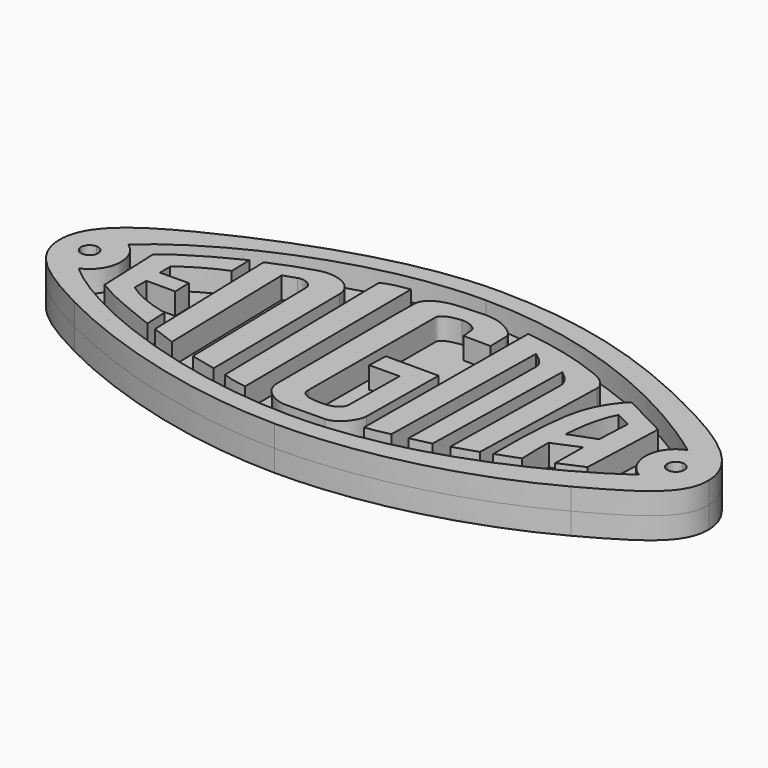
from build123d import *

# Parameters (mm, degrees)
F1_DEPTH = 1
F2_DEPTH = 1


# Not quite as in the source:
# - ends of sketch curves that miss each other by under 0.0002 mm in the source are joined


with BuildPart() as f1:
    # F0 (on Top) → F1 (new body)
    with BuildSketch(Plane.XY):
        with BuildLine():
            add(Edge.make_bspline(
                [(-14.9670643715, -0.1407183656), (-14.9569619615, 1.2571726483), (-13.641275343, 2.2858408304), (-11.5509025419, 3.3477109063)],
                knots=[0, 0, 0, 0, 1, 1, 1, 1], degree=3))
            add(Edge.make_bspline(
                [(-11.5044687858, -3.6532307803), (-13.8905338724, -2.4348834013), (-14.9771667815, -1.5386093795), (-14.9670643715, -0.1407183656)],
                knots=[0, 0, 0, 0, 1, 1, 1, 1], degree=3))
            add(Edge.make_bspline(
                [(0.0408589419, -6.5594502425), (-4.0268959211, -6.5322608085), (-8.2906712355, -5.2942260219), (-11.5044687858, -3.6532307803)],
                knots=[0, 0, 0, 0, 1, 1, 1, 1], degree=3))
            add(Edge.make_bspline(
                [(11.460803766, -3.7191493993), (8.3259909371, -5.4149417683), (4.1086135021, -6.5866396765), (0.0408589419, -6.5594502425)],
                knots=[0, 0, 0, 0, 1, 1, 1, 1], degree=3))
            add(Edge.make_bspline(
                [(15.0329356285, -0.2313463811), (15.0665385246, -1.6458235069), (13.7252402924, -2.4941911604), (11.460803766, -3.7191493993)],
                knots=[0, 0, 0, 0, 1, 1, 1, 1], degree=3))
            add(Edge.make_bspline(
                [(11.5176890114, 3.3904380032), (13.5946130245, 2.2916362132), (14.9993327324, 1.1831307446), (15.0329356285, -0.2313463811)],
                knots=[0, 0, 0, 0, 1, 1, 1, 1], degree=3))
            add(Edge.make_bspline(
                [(0.0012151267, 6.5835113531), (4.2558432307, 6.5477381404), (7.5924313242, 5.4671057322), (11.5176890114, 3.3904380032)],
                knots=[0, 0, 0, 0, 1, 1, 1, 1], degree=3))
            add(Edge.make_bspline(
                [(-11.5509025419, 3.3477109063), (-8.7841304286, 4.7531791819), (-4.2534132801, 6.6192845659), (0.0012151267, 6.5835113531)],
                knots=[0, 0, 0, 0, 1, 1, 1, 1], degree=3))
        make_face()
        with BuildLine():
            add(Edge.make_bspline(
                [(-13.6112109244, 0.2440781572), (-13.3944005743, 0.2441072219), (-13.2186146132, 0.0683763627), (-13.2185758603, -0.1484339874)],
                knots=[0, 0, 0, 0, 1, 1, 1, 1], degree=3))
            add(Edge.make_bspline(
                [(-13.2185758603, -0.1484339874), (-13.2185758603, -0.3653145773), (-13.3943303345, -0.5410769233), (-13.6111406847, -0.5410866115)],
                knots=[0, 0, 0, 0, 1, 1, 1, 1], degree=3))
            add(Edge.make_bspline(
                [(-13.6111406847, -0.5410866115), (-13.8279511862, -0.5410962997), (-14.0037212525, -0.3653498485), (-14.0037407803, -0.148539347)],
                knots=[0, 0, 0, 0, 1, 1, 1, 1], degree=3))
            add(Edge.make_bspline(
                [(-14.0037407803, -0.148539347), (-14.0037601568, 0.0682710031), (-13.8280214259, 0.2440490925), (-13.6112109244, 0.2440781572)],
                knots=[0, 0, 0, 0, 1, 1, 1, 1], degree=3))
        make_face(mode=Mode.SUBTRACT)
        with BuildLine():
            add(Edge.make_bspline(
                [(-0.0131874985, -5.7002234367), (-5.2648230774, -5.6636889404), (-10.8317908165, -3.4899332606), (-13.0370717195, -1.5029596918)],
                knots=[0, 0, 0, 0, 1, 1, 1, 1], degree=3))
            add(Edge.make_bspline(
                [(-13.0370717195, -1.5029596918), (-11.9503426849, -1.0492089526), (-11.8638049223, 0.4456897815), (-12.8094284057, 1.0703302885)],
                knots=[0, 0, 0, 0, 1, 1, 1, 1], degree=3))
            add(Edge.make_bspline(
                [(-12.8094284057, 1.0703302885), (-10.2644291395, 3.343872699), (-5.0939152955, 5.7284840957), (-0.0131874985, 5.7189015202)],
                knots=[0, 0, 0, 0, 1, 1, 1, 1], degree=3))
            add(Edge.make_bspline(
                [(-0.0131874985, 5.7189015202), (5.0675404498, 5.7093187933), (9.7327737855, 3.5101702421), (12.9692698175, 1.1270839859)],
                knots=[0, 0, 0, 0, 1, 1, 1, 1], degree=3))
            add(Edge.make_bspline(
                [(12.9692698175, 1.1270839859), (11.7931722383, 0.6908568469), (11.801028945, -0.9240995903), (12.8031188089, -1.4633658316)],
                knots=[0, 0, 0, 0, 1, 1, 1, 1], degree=3))
            add(Edge.make_bspline(
                [(12.8031188089, -1.4633658316), (10.1548959098, -3.3464114023), (5.2384480804, -5.7367579331), (-0.0131874985, -5.7002234367)],
                knots=[0, 0, 0, 0, 1, 1, 1, 1], degree=3))
        make_face(mode=Mode.SUBTRACT)
        with BuildLine():
            add(Edge.make_bspline(
                [(13.4484099464, 0.2319138177), (13.6652202965, 0.2319430338), (13.8410062576, 0.0562121746), (13.8410450105, -0.1605983269)],
                knots=[0, 0, 0, 0, 1, 1, 1, 1], degree=3))
            add(Edge.make_bspline(
                [(13.8410450105, -0.1605983269), (13.8410450105, -0.3774789168), (13.6652905362, -0.5532412628), (13.4484801861, -0.553250951)],
                knots=[0, 0, 0, 0, 1, 1, 1, 1], degree=3))
            add(Edge.make_bspline(
                [(13.4484801861, -0.553250951), (13.231669836, -0.5532606393), (13.0558996183, -0.3775140367), (13.0558802418, -0.1607036865)],
                knots=[0, 0, 0, 0, 1, 1, 1, 1], degree=3))
            add(Edge.make_bspline(
                [(13.0558802418, -0.1607036865), (13.055860714, 0.0561066636), (13.2315994449, 0.231884753), (13.4484099464, 0.2319138177)],
                knots=[0, 0, 0, 0, 1, 1, 1, 1], degree=3))
        make_face(mode=Mode.SUBTRACT)
    extrude(amount=F1_DEPTH)


with BuildPart() as f1b:
    # F0 (on Top) → F1, piece 2 (new body)
    with BuildSketch(Plane.XY):
        with BuildLine():
            Line((-11.6211207706, 1.0289036862), (-11.5002833157, -1.9165056063))
            add(Edge.make_bspline(
                [(-11.5002833157, -1.9165056063), (-10.5464697896, -2.5212275505), (-9.4578547276, -2.8833071235), (-8.4113801698, -3.3212389382)],
                knots=[0, 0, 0, 0, 1, 1, 1, 1], degree=3))
            Line((-8.4113801698, -3.3212389382), (-8.4566941776, -2.27146493))
            add(Edge.make_bspline(
                [(-8.4566941776, -2.27146493), (-9.605320607, -2.0319305152), (-10.5260527366, -1.4709255333), (-10.5260327546, -1.3651853806)],
                knots=[0, 0, 0, 0, 1, 1, 1, 1], degree=3))
            Line((-10.5260327546, -1.3651853806), (-10.5184803191, -0.7383417077))
            Line((-10.5184803191, -0.7383417077), (-9.189270283, -0.7383417077))
            Line((-9.189270283, -0.7383417077), (-9.2119272868, 0.0773099777))
            Line((-9.2119272868, 0.0773099777), (-10.5335851902, 0.0622055607))
            Line((-10.5335851902, 0.0622055607), (-10.5411371716, 0.6437347718))
            add(Edge.make_bspline(
                [(-10.5411371716, 0.6437347718), (-10.5413080782, 0.7288635012), (-9.4660527933, 1.4647343644), (-8.6001881822, 1.7841367955)],
                knots=[0, 0, 0, 0, 1, 1, 1, 1], degree=3))
            Line((-8.6001881822, 1.7841367955), (-8.6228450347, 2.8414632393))
            add(Edge.make_bspline(
                [(-8.6228450347, 2.8414632393), (-9.5944114998, 2.3620312522), (-10.7739830692, 1.7207511966), (-11.6211207706, 1.0289036862)],
                knots=[0, 0, 0, 0, 1, 1, 1, 1], degree=3))
        make_face()
    extrude(amount=F1_DEPTH)


with BuildPart() as f1c:
    # F0 (on Top) → F1, piece 3 (new body)
    with BuildSketch(Plane.XY):
        with BuildLine():
            Line((-4.3633304258, -4.5522689775), (-4.4388534188, 2.788596796))
            add(Edge.make_bspline(
                [(-4.4388534188, 2.788596796), (-4.4690630096, 3.6797719285), (-5.5116984517, 3.9135012722), (-6.100366683, 3.7704002467)],
                knots=[0, 0, 0, 0, 1, 1, 1, 1], degree=3))
            add(Edge.make_bspline(
                [(-8.1243912523, 3.0302717058), (-7.7536792271, 3.1870081507), (-7.0454069014, 3.486464545), (-6.4053945164, 3.6787551609), (-6.100366683, 3.7704002467)],
                knots=[0, 0, 0, 0, 0.5234032331, 1, 1, 1, 1], degree=3))
            Line((-8.1243912523, 3.0302717058), (-7.9280308043, -3.4798379654))
            Line((-7.9280308043, -3.4798379654), (-6.8253903528, -3.8876641865))
            Line((-6.8253903528, -3.8876641865), (-6.976436793, 2.6375503558))
            Line((-6.976436793, 2.6375503558), (-6.4024595634, 2.8339108037))
            add(Edge.make_bspline(
                [(-6.4024595634, 2.8339108037), (-6.1154712513, 2.9396436903), (-5.707645333, 2.7281783713), (-5.692540916, 2.4713988931)],
                knots=[0, 0, 0, 0, 1, 1, 1, 1], degree=3))
            Line((-5.692540916, 2.4713988931), (-5.5414940217, -4.2803850824))
            Line((-5.5414940217, -4.2803850824), (-4.3633304258, -4.5522689775))
        make_face()
    extrude(amount=F1_DEPTH)


with BuildPart() as f1d:
    # F0 (on Top) → F1, piece 4 (new body)
    with BuildSketch(Plane.XY):
        with BuildLine():
            Line((-2.5960847291, -4.9449901761), (-2.6565033052, 4.6917845159))
            add(Edge.make_bspline(
                [(-2.6565033052, 4.6917845159), (-3.0422194537, 4.6081617018), (-3.313422296, 4.6390521941), (-3.8799812116, 4.374586613)],
                knots=[0, 0, 0, 0, 1, 1, 1, 1], degree=3))
            Line((-3.8799812116, 4.374586613), (-3.7289343173, -4.6882113035))
            add(Edge.make_bspline(
                [(-3.7289343173, -4.6882113035), (-3.2986876972, -4.852749069), (-2.9477797221, -4.8982792456), (-2.5960847291, -4.9449901761)],
                knots=[0, 0, 0, 0, 1, 1, 1, 1], degree=3))
        make_face()
    extrude(amount=F1_DEPTH)


with BuildPart() as f1e:
    # F0 (on Top) → F1, piece 5 (new body)
    with BuildSketch(Plane.XY):
        with BuildLine():
            Line((1.2556039615, -0.8516265756), (1.2253949763, -3.6913037385))
            add(Edge.make_bspline(
                [(1.2253949763, -3.6913037385), (1.2253945221, -3.9782917478), (1.0288969251, -4.2504746159), (0.3191149727, -4.2501756429)],
                knots=[0, 0, 0, 0, 1, 1, 1, 1], degree=3))
            add(Edge.make_bspline(
                [(0.3191149727, -4.2501756429), (-0.4969122832, -4.2498338298), (-0.6475831528, -4.0085011873), (-0.6324787359, -3.7366172921)],
                knots=[0, 0, 0, 0, 1, 1, 1, 1], degree=3))
            add(Edge.make_bspline(
                [(-0.6324787359, -3.7366172921), (-0.6173741676, -3.464733397), (-0.6022691451, 3.2719461615), (-0.6022691451, 3.5438299052)],
                knots=[0, 0, 0, 0, 1, 1, 1, 1], degree=3))
            add(Edge.make_bspline(
                [(-0.6022691451, 3.5438299052), (-0.6022691451, 3.8157138003), (-0.0433969379, 3.9516558236), (0.288905836, 3.9667606946)],
                knots=[0, 0, 0, 0, 1, 1, 1, 1], degree=3))
            add(Edge.make_bspline(
                [(0.288905836, 3.9667606946), (0.6212083072, 3.981865263), (1.0441390966, 3.7724048037), (1.0441390966, 3.5438299052)],
                knots=[0, 0, 0, 0, 1, 1, 1, 1], degree=3))
            Line((1.0441390966, 3.5438299052), (1.089452953, 3.0453761227))
            Line((1.089452953, 3.0453761227), (2.3431399961, 3.0302717058))
            Line((2.3431399961, 3.0302717058), (2.3280349736, 3.9516558236))
            add(Edge.make_bspline(
                [(2.3280349736, 3.9516558236), (2.3129305567, 4.2839585975), (1.6030113038, 4.7068889328), (1.089452953, 4.78241238)],
                knots=[0, 0, 0, 0, 1, 1, 1, 1], degree=3))
            add(Edge.make_bspline(
                [(1.089452953, 4.78241238), (0.5758942995, 4.8579358271), (0.54568486, 4.78241238), (-0.2699668253, 4.767307963)],
                knots=[0, 0, 0, 0, 1, 1, 1, 1], degree=3))
            add(Edge.make_bspline(
                [(-0.2699668253, 4.767307963), (-1.0856185106, 4.7522029406), (-1.7955376121, 4.4803190454), (-1.8559561882, 3.9365512552)],
                knots=[0, 0, 0, 0, 1, 1, 1, 1], degree=3))
            add(Edge.make_bspline(
                [(-1.8559561882, 3.9365512552), (-1.916375067, 3.392783465), (-1.8106421804, -3.4345239576), (-1.8408516199, -4.053815195)],
                knots=[0, 0, 0, 0, 1, 1, 1, 1], degree=3))
            add(Edge.make_bspline(
                [(-1.8408516199, -4.053815195), (-1.8710610593, -4.673106281), (-1.1007233817, -5.1564556465), (-0.5871647281, -5.1564556465)],
                knots=[0, 0, 0, 0, 1, 1, 1, 1], degree=3))
            add(Edge.make_bspline(
                [(-0.5871647281, -5.1564556465), (-0.0736059232, -5.1564556465), (0.6967317544, -5.1564556465), (1.2556039615, -5.1413510782)],
                knots=[0, 0, 0, 0, 1, 1, 1, 1], degree=3))
            add(Edge.make_bspline(
                [(1.2556039615, -5.1413510782), (1.8144767742, -5.1262462071), (2.2676165489, -4.4465363936), (2.2827211173, -4.0387106267)],
                knots=[0, 0, 0, 0, 1, 1, 1, 1], degree=3))
            Line((2.2827211173, -4.0387106267), (2.3280349736, 0.0546529738))
            Line((2.3280349736, 0.0546529738), (-0.1038153626, 0.0546529738))
            Line((-0.1038153626, 0.0546529738), (-0.1340249534, -0.8667315981))
            Line((-0.1340249534, -0.8667315981), (1.2556039615, -0.8516265756))
        make_face()
    extrude(amount=F1_DEPTH)


with BuildPart() as f1f:
    # F0 (on Top) → F1, piece 6 (new body)
    with BuildSketch(Plane.XY):
        with BuildLine():
            Line((7.2068412741, -3.661093845), (7.4032021762, 2.849015372))
            add(Edge.make_bspline(
                [(7.4032021762, 2.849015372), (7.4183067446, 3.1511087066), (7.049798723, 3.505934817), (6.5875500368, 3.6797719285)],
                knots=[0, 0, 0, 0, 1, 1, 1, 1], degree=3))
            ThreePointArc((6.5875500368, 3.6797719285), (4.731040618, 4.2753288203), (2.8113843392, 4.6162613714))
            Line((2.8113843392, 4.6162613714), (2.7509657631, -4.778839319))
            add(Edge.make_bspline(
                [(2.7509657631, -4.778839319), (3.1297758632, -4.7196140613), (3.5135646579, -4.6653676496), (3.8536062146, -4.5673738486)],
                knots=[0, 0, 0, 0, 1, 1, 1, 1], degree=3))
            Line((3.8536062146, -4.5673738486), (4.0046528062, 3.5891443671))
            add(Edge.make_bspline(
                [(4.0046528062, 3.5891443671), (4.0720203225, 3.5379805902), (4.1828123319, 3.4522951468), (4.2144659213, 3.4274451231), (4.2906508935, 3.3664320253), (4.4687473777, 3.2021661464), (4.6033155082, 2.9884969513), (4.6326551395, 2.8839476867), (4.6373056055, 2.824720552), (4.6390484605, 2.8037018184)],
                knots=[0, 0, 0, 0, 0.1850054035, 0.2612916033, 0.3753300897, 0.5703100306, 0.7666527828, 0.8936191452, 1, 1, 1, 1], degree=3))
            Line((4.6390484605, 2.8037018184), (4.5333160281, -4.4314319767))
            add(Edge.make_bspline(
                [(4.5333160281, -4.4314319767), (4.8354789968, -4.3709433123), (5.1293064479, -4.318790771), (5.4698050169, -4.2199665063)],
                knots=[0, 0, 0, 0, 1, 1, 1, 1], degree=3))
            Line((5.4698050169, -4.2199665063), (5.6359564796, 3.0604806911))
            add(Edge.make_bspline(
                [(5.6359564796, 3.0604806911), (5.785887239, 2.9409553318), (6.0576444833, 2.7243094457), (6.2258203773, 2.3756907044), (6.2361157634, 2.2599070967), (6.2401426945, 2.2146195663)],
                knots=[0, 0, 0, 0, 0.4283490631, 0.7764047978, 1, 1, 1, 1], degree=3))
            Line((6.2401426945, 2.2146195663), (6.119305391, -4.0085011873))
            add(Edge.make_bspline(
                [(6.119305391, -4.0085011873), (6.4699454257, -3.904570767), (6.817240445, -3.8039850596), (7.2068412741, -3.661093845)],
                knots=[0, 0, 0, 0, 1, 1, 1, 1], degree=3))
        make_face()
    extrude(amount=F1_DEPTH)


with BuildPart() as f1g:
    # F0 (on Top) → F1, piece 7 (new body)
    with BuildSketch(Plane.XY):
        with BuildLine():
            Line((9.8671853699, -2.6448491628), (10.9779687853, -2.164221738))
            Line((10.9779687853, -2.164221738), (11.1274973511, 1.7128389338))
            Line((11.1274973511, 1.7128389338), (9.055459086, 2.7808999451))
            add(Edge.make_bspline(
                [(7.6776605692, -3.4779368001), (7.6761910448, -2.9670023712), (7.6730666864, -1.8807037051), (7.7992836376, 0.1813668207), (8.0436769948, 1.2326744215), (8.4274407257, 2.0619125257), (8.9246206003, 2.6759028048), (9.0247880348, 2.756286601), (9.055459086, 2.7808999451)],
                knots=[0, 0, 0, 0, 0.2136285367, 0.4541960402, 0.628207252, 0.7899148708, 0.935672389, 1, 1, 1, 1], degree=3))
            Line((7.6776605692, -3.4779368001), (8.7136795503, -3.1041153856))
            add(Edge.make_bspline(
                [(8.7136795503, -3.1041153856), (8.7045593073, -2.8555582906), (8.6868684619, -2.3734236481), (8.6852845097, -1.6678730588), (8.6948580771, -1.5618086592), (8.7015062661, -1.5565972505), (8.702999025, -1.5554271008)],
                knots=[0, 0, 0, 0, 0.4262627423, 0.8268363249, 0.9611184917, 1, 1, 1, 1], degree=3))
            Line((8.702999025, -1.5554271008), (9.8885467233, -1.0534384739))
            Line((9.8885467233, -1.0534384739), (9.8671853699, -2.6448491628))
        make_face()
        with BuildLine():
            add(Edge.make_bspline(
                [(9.3011131368, 1.7235196105), (8.9318485244, 0.9931556023), (8.8098038243, 0.1356684408), (8.7564021058, -0.6475751806)],
                knots=[0, 0, 0, 0, 1, 1, 1, 1], degree=3))
            Line((9.3011131368, 1.7235196105), (10.0167139357, 1.3603788727))
            Line((10.0167139357, 1.3603788727), (9.9419496528, -0.1989896346))
            Line((9.9419496528, -0.1989896346), (8.7564021058, -0.6475751806))
        make_face(mode=Mode.SUBTRACT)
    extrude(amount=F1_DEPTH)


with BuildPart() as f2:
    # F0 (on Top) → F2 (new body)
    with BuildSketch(Plane.XY):
        with BuildLine():
            add(Edge.make_bspline(
                [(-14.9670643715, -0.1407183656), (-14.9569619615, 1.2571726483), (-13.641275343, 2.2858408304), (-11.5509025419, 3.3477109063)],
                knots=[0, 0, 0, 0, 1, 1, 1, 1], degree=3))
            add(Edge.make_bspline(
                [(-11.5044687858, -3.6532307803), (-13.8905338724, -2.4348834013), (-14.9771667815, -1.5386093795), (-14.9670643715, -0.1407183656)],
                knots=[0, 0, 0, 0, 1, 1, 1, 1], degree=3))
            add(Edge.make_bspline(
                [(0.0408589419, -6.5594502425), (-4.0268959211, -6.5322608085), (-8.2906712355, -5.2942260219), (-11.5044687858, -3.6532307803)],
                knots=[0, 0, 0, 0, 1, 1, 1, 1], degree=3))
            add(Edge.make_bspline(
                [(11.460803766, -3.7191493993), (8.3259909371, -5.4149417683), (4.1086135021, -6.5866396765), (0.0408589419, -6.5594502425)],
                knots=[0, 0, 0, 0, 1, 1, 1, 1], degree=3))
            add(Edge.make_bspline(
                [(15.0329356285, -0.2313463811), (15.0665385246, -1.6458235069), (13.7252402924, -2.4941911604), (11.460803766, -3.7191493993)],
                knots=[0, 0, 0, 0, 1, 1, 1, 1], degree=3))
            add(Edge.make_bspline(
                [(11.5176890114, 3.3904380032), (13.5946130245, 2.2916362132), (14.9993327324, 1.1831307446), (15.0329356285, -0.2313463811)],
                knots=[0, 0, 0, 0, 1, 1, 1, 1], degree=3))
            add(Edge.make_bspline(
                [(0.0012151267, 6.5835113531), (4.2558432307, 6.5477381404), (7.5924313242, 5.4671057322), (11.5176890114, 3.3904380032)],
                knots=[0, 0, 0, 0, 1, 1, 1, 1], degree=3))
            add(Edge.make_bspline(
                [(-11.5509025419, 3.3477109063), (-8.7841304286, 4.7531791819), (-4.2534132801, 6.6192845659), (0.0012151267, 6.5835113531)],
                knots=[0, 0, 0, 0, 1, 1, 1, 1], degree=3))
        make_face()
        with BuildLine():
            add(Edge.make_bspline(
                [(-13.6112109244, 0.2440781572), (-13.3944005743, 0.2441072219), (-13.2186146132, 0.0683763627), (-13.2185758603, -0.1484339874)],
                knots=[0, 0, 0, 0, 1, 1, 1, 1], degree=3))
            add(Edge.make_bspline(
                [(-13.2185758603, -0.1484339874), (-13.2185758603, -0.3653145773), (-13.3943303345, -0.5410769233), (-13.6111406847, -0.5410866115)],
                knots=[0, 0, 0, 0, 1, 1, 1, 1], degree=3))
            add(Edge.make_bspline(
                [(-13.6111406847, -0.5410866115), (-13.8279511862, -0.5410962997), (-14.0037212525, -0.3653498485), (-14.0037407803, -0.148539347)],
                knots=[0, 0, 0, 0, 1, 1, 1, 1], degree=3))
            add(Edge.make_bspline(
                [(-14.0037407803, -0.148539347), (-14.0037601568, 0.0682710031), (-13.8280214259, 0.2440490925), (-13.6112109244, 0.2440781572)],
                knots=[0, 0, 0, 0, 1, 1, 1, 1], degree=3))
        make_face(mode=Mode.SUBTRACT)
        with BuildLine():
            add(Edge.make_bspline(
                [(-0.0131874985, -5.7002234367), (-5.2648230774, -5.6636889404), (-10.8317908165, -3.4899332606), (-13.0370717195, -1.5029596918)],
                knots=[0, 0, 0, 0, 1, 1, 1, 1], degree=3))
            add(Edge.make_bspline(
                [(-13.0370717195, -1.5029596918), (-11.9503426849, -1.0492089526), (-11.8638049223, 0.4456897815), (-12.8094284057, 1.0703302885)],
                knots=[0, 0, 0, 0, 1, 1, 1, 1], degree=3))
            add(Edge.make_bspline(
                [(-12.8094284057, 1.0703302885), (-10.2644291395, 3.343872699), (-5.0939152955, 5.7284840957), (-0.0131874985, 5.7189015202)],
                knots=[0, 0, 0, 0, 1, 1, 1, 1], degree=3))
            add(Edge.make_bspline(
                [(-0.0131874985, 5.7189015202), (5.0675404498, 5.7093187933), (9.7327737855, 3.5101702421), (12.9692698175, 1.1270839859)],
                knots=[0, 0, 0, 0, 1, 1, 1, 1], degree=3))
            add(Edge.make_bspline(
                [(12.9692698175, 1.1270839859), (11.7931722383, 0.6908568469), (11.801028945, -0.9240995903), (12.8031188089, -1.4633658316)],
                knots=[0, 0, 0, 0, 1, 1, 1, 1], degree=3))
            add(Edge.make_bspline(
                [(12.8031188089, -1.4633658316), (10.1548959098, -3.3464114023), (5.2384480804, -5.7367579331), (-0.0131874985, -5.7002234367)],
                knots=[0, 0, 0, 0, 1, 1, 1, 1], degree=3))
        make_face(mode=Mode.SUBTRACT)
        with BuildLine():
            add(Edge.make_bspline(
                [(13.4484099464, 0.2319138177), (13.6652202965, 0.2319430338), (13.8410062576, 0.0562121746), (13.8410450105, -0.1605983269)],
                knots=[0, 0, 0, 0, 1, 1, 1, 1], degree=3))
            add(Edge.make_bspline(
                [(13.8410450105, -0.1605983269), (13.8410450105, -0.3774789168), (13.6652905362, -0.5532412628), (13.4484801861, -0.553250951)],
                knots=[0, 0, 0, 0, 1, 1, 1, 1], degree=3))
            add(Edge.make_bspline(
                [(13.4484801861, -0.553250951), (13.231669836, -0.5532606393), (13.0558996183, -0.3775140367), (13.0558802418, -0.1607036865)],
                knots=[0, 0, 0, 0, 1, 1, 1, 1], degree=3))
            add(Edge.make_bspline(
                [(13.0558802418, -0.1607036865), (13.055860714, 0.0561066636), (13.2315994449, 0.231884753), (13.4484099464, 0.2319138177)],
                knots=[0, 0, 0, 0, 1, 1, 1, 1], degree=3))
        make_face(mode=Mode.SUBTRACT)
        with BuildLine():
            add(Edge.make_bspline(
                [(-13.0370717195, -1.5029596918), (-11.9503426849, -1.0492089526), (-11.8638049223, 0.4456897815), (-12.8094284057, 1.0703302885)],
                knots=[0, 0, 0, 0, 1, 1, 1, 1], degree=3))
            add(Edge.make_bspline(
                [(-0.0131874985, -5.7002234367), (-5.2648230774, -5.6636889404), (-10.8317908165, -3.4899332606), (-13.0370717195, -1.5029596918)],
                knots=[0, 0, 0, 0, 1, 1, 1, 1], degree=3))
            add(Edge.make_bspline(
                [(12.8031188089, -1.4633658316), (10.1548959098, -3.3464114023), (5.2384480804, -5.7367579331), (-0.0131874985, -5.7002234367)],
                knots=[0, 0, 0, 0, 1, 1, 1, 1], degree=3))
            add(Edge.make_bspline(
                [(12.9692698175, 1.1270839859), (11.7931722383, 0.6908568469), (11.801028945, -0.9240995903), (12.8031188089, -1.4633658316)],
                knots=[0, 0, 0, 0, 1, 1, 1, 1], degree=3))
            add(Edge.make_bspline(
                [(-0.0131874985, 5.7189015202), (5.0675404498, 5.7093187933), (9.7327737855, 3.5101702421), (12.9692698175, 1.1270839859)],
                knots=[0, 0, 0, 0, 1, 1, 1, 1], degree=3))
            add(Edge.make_bspline(
                [(-12.8094284057, 1.0703302885), (-10.2644291395, 3.343872699), (-5.0939152955, 5.7284840957), (-0.0131874985, 5.7189015202)],
                knots=[0, 0, 0, 0, 1, 1, 1, 1], degree=3))
        make_face()
        with BuildLine():
            add(Edge.make_bspline(
                [(-11.5002833157, -1.9165056063), (-10.5464697896, -2.5212275505), (-9.4578547276, -2.8833071235), (-8.4113801698, -3.3212389382)],
                knots=[0, 0, 0, 0, 1, 1, 1, 1], degree=3))
            Line((-11.5002833157, -1.9165056063), (-11.6211207706, 1.0289036862))
            add(Edge.make_bspline(
                [(-8.6228450347, 2.8414632393), (-9.5944114998, 2.3620312522), (-10.7739830692, 1.7207511966), (-11.6211207706, 1.0289036862)],
                knots=[0, 0, 0, 0, 1, 1, 1, 1], degree=3))
            Line((-8.6228450347, 2.8414632393), (-8.6001881822, 1.7841367955))
            add(Edge.make_bspline(
                [(-10.5411371716, 0.6437347718), (-10.5413080782, 0.7288635012), (-9.4660527933, 1.4647343644), (-8.6001881822, 1.7841367955)],
                knots=[0, 0, 0, 0, 1, 1, 1, 1], degree=3))
            Line((-10.5411371716, 0.6437347718), (-10.5335851902, 0.0622055607))
            Line((-10.5335851902, 0.0622055607), (-9.2119272868, 0.0773099777))
            Line((-9.2119272868, 0.0773099777), (-9.189270283, -0.7383417077))
            Line((-9.189270283, -0.7383417077), (-10.5184803191, -0.7383417077))
            Line((-10.5184803191, -0.7383417077), (-10.5260327546, -1.3651853806))
            add(Edge.make_bspline(
                [(-8.4566941776, -2.27146493), (-9.605320607, -2.0319305152), (-10.5260527366, -1.4709255333), (-10.5260327546, -1.3651853806)],
                knots=[0, 0, 0, 0, 1, 1, 1, 1], degree=3))
            Line((-8.4566941776, -2.27146493), (-8.4113801698, -3.3212389382))
        make_face(mode=Mode.SUBTRACT)
        with BuildLine():
            add(Edge.make_bspline(
                [(-4.4388534188, 2.788596796), (-4.4690630096, 3.6797719285), (-5.5116984517, 3.9135012722), (-6.100366683, 3.7704002467)],
                knots=[0, 0, 0, 0, 1, 1, 1, 1], degree=3))
            Line((-4.4388534188, 2.788596796), (-4.3633304258, -4.5522689775))
            Line((-4.3633304258, -4.5522689775), (-5.5414940217, -4.2803850824))
            Line((-5.5414940217, -4.2803850824), (-5.692540916, 2.4713988931))
            add(Edge.make_bspline(
                [(-6.4024595634, 2.8339108037), (-6.1154712513, 2.9396436903), (-5.707645333, 2.7281783713), (-5.692540916, 2.4713988931)],
                knots=[0, 0, 0, 0, 1, 1, 1, 1], degree=3))
            Line((-6.4024595634, 2.8339108037), (-6.976436793, 2.6375503558))
            Line((-6.976436793, 2.6375503558), (-6.8253903528, -3.8876641865))
            Line((-6.8253903528, -3.8876641865), (-7.9280308043, -3.4798379654))
            Line((-7.9280308043, -3.4798379654), (-8.1243912523, 3.0302717058))
            add(Edge.make_bspline(
                [(-8.1243912523, 3.0302717058), (-7.7536792271, 3.1870081507), (-7.0454069014, 3.486464545), (-6.4053945164, 3.6787551609), (-6.100366683, 3.7704002467)],
                knots=[0, 0, 0, 0, 0.5234032331, 1, 1, 1, 1], degree=3))
        make_face(mode=Mode.SUBTRACT)
        with BuildLine():
            add(Edge.make_bspline(
                [(-2.6565033052, 4.6917845159), (-3.0422194537, 4.6081617018), (-3.313422296, 4.6390521941), (-3.8799812116, 4.374586613)],
                knots=[0, 0, 0, 0, 1, 1, 1, 1], degree=3))
            Line((-2.6565033052, 4.6917845159), (-2.5960847291, -4.9449901761))
            add(Edge.make_bspline(
                [(-3.7289343173, -4.6882113035), (-3.2986876972, -4.852749069), (-2.9477797221, -4.8982792456), (-2.5960847291, -4.9449901761)],
                knots=[0, 0, 0, 0, 1, 1, 1, 1], degree=3))
            Line((-3.7289343173, -4.6882113035), (-3.8799812116, 4.374586613))
        make_face(mode=Mode.SUBTRACT)
        with BuildLine():
            add(Edge.make_bspline(
                [(1.2253949763, -3.6913037385), (1.2253945221, -3.9782917478), (1.0288969251, -4.2504746159), (0.3191149727, -4.2501756429)],
                knots=[0, 0, 0, 0, 1, 1, 1, 1], degree=3))
            Line((1.2253949763, -3.6913037385), (1.2556039615, -0.8516265756))
            Line((1.2556039615, -0.8516265756), (-0.1340249534, -0.8667315981))
            Line((-0.1340249534, -0.8667315981), (-0.1038153626, 0.0546529738))
            Line((-0.1038153626, 0.0546529738), (2.3280349736, 0.0546529738))
            Line((2.3280349736, 0.0546529738), (2.2827211173, -4.0387106267))
            add(Edge.make_bspline(
                [(1.2556039615, -5.1413510782), (1.8144767742, -5.1262462071), (2.2676165489, -4.4465363936), (2.2827211173, -4.0387106267)],
                knots=[0, 0, 0, 0, 1, 1, 1, 1], degree=3))
            add(Edge.make_bspline(
                [(-0.5871647281, -5.1564556465), (-0.0736059232, -5.1564556465), (0.6967317544, -5.1564556465), (1.2556039615, -5.1413510782)],
                knots=[0, 0, 0, 0, 1, 1, 1, 1], degree=3))
            add(Edge.make_bspline(
                [(-1.8408516199, -4.053815195), (-1.8710610593, -4.673106281), (-1.1007233817, -5.1564556465), (-0.5871647281, -5.1564556465)],
                knots=[0, 0, 0, 0, 1, 1, 1, 1], degree=3))
            add(Edge.make_bspline(
                [(-1.8559561882, 3.9365512552), (-1.916375067, 3.392783465), (-1.8106421804, -3.4345239576), (-1.8408516199, -4.053815195)],
                knots=[0, 0, 0, 0, 1, 1, 1, 1], degree=3))
            add(Edge.make_bspline(
                [(-0.2699668253, 4.767307963), (-1.0856185106, 4.7522029406), (-1.7955376121, 4.4803190454), (-1.8559561882, 3.9365512552)],
                knots=[0, 0, 0, 0, 1, 1, 1, 1], degree=3))
            add(Edge.make_bspline(
                [(1.089452953, 4.78241238), (0.5758942995, 4.8579358271), (0.54568486, 4.78241238), (-0.2699668253, 4.767307963)],
                knots=[0, 0, 0, 0, 1, 1, 1, 1], degree=3))
            add(Edge.make_bspline(
                [(2.3280349736, 3.9516558236), (2.3129305567, 4.2839585975), (1.6030113038, 4.7068889328), (1.089452953, 4.78241238)],
                knots=[0, 0, 0, 0, 1, 1, 1, 1], degree=3))
            Line((2.3280349736, 3.9516558236), (2.3431399961, 3.0302717058))
            Line((2.3431399961, 3.0302717058), (1.089452953, 3.0453761227))
            Line((1.089452953, 3.0453761227), (1.0441390966, 3.5438299052))
            add(Edge.make_bspline(
                [(0.288905836, 3.9667606946), (0.6212083072, 3.981865263), (1.0441390966, 3.7724048037), (1.0441390966, 3.5438299052)],
                knots=[0, 0, 0, 0, 1, 1, 1, 1], degree=3))
            add(Edge.make_bspline(
                [(-0.6022691451, 3.5438299052), (-0.6022691451, 3.8157138003), (-0.0433969379, 3.9516558236), (0.288905836, 3.9667606946)],
                knots=[0, 0, 0, 0, 1, 1, 1, 1], degree=3))
            add(Edge.make_bspline(
                [(-0.6324787359, -3.7366172921), (-0.6173741676, -3.464733397), (-0.6022691451, 3.2719461615), (-0.6022691451, 3.5438299052)],
                knots=[0, 0, 0, 0, 1, 1, 1, 1], degree=3))
            add(Edge.make_bspline(
                [(0.3191149727, -4.2501756429), (-0.4969122832, -4.2498338298), (-0.6475831528, -4.0085011873), (-0.6324787359, -3.7366172921)],
                knots=[0, 0, 0, 0, 1, 1, 1, 1], degree=3))
        make_face(mode=Mode.SUBTRACT)
        with BuildLine():
            add(Edge.make_bspline(
                [(7.4032021762, 2.849015372), (7.4183067446, 3.1511087066), (7.049798723, 3.505934817), (6.5875500368, 3.6797719285)],
                knots=[0, 0, 0, 0, 1, 1, 1, 1], degree=3))
            Line((7.4032021762, 2.849015372), (7.2068412741, -3.661093845))
            add(Edge.make_bspline(
                [(6.119305391, -4.0085011873), (6.4699454257, -3.904570767), (6.817240445, -3.8039850596), (7.2068412741, -3.661093845)],
                knots=[0, 0, 0, 0, 1, 1, 1, 1], degree=3))
            Line((6.119305391, -4.0085011873), (6.2401426945, 2.2146195663))
            add(Edge.make_bspline(
                [(5.6359564796, 3.0604806911), (5.785887239, 2.9409553318), (6.0576444833, 2.7243094457), (6.2258203773, 2.3756907044), (6.2361157634, 2.2599070967), (6.2401426945, 2.2146195663)],
                knots=[0, 0, 0, 0, 0.4283490631, 0.7764047978, 1, 1, 1, 1], degree=3))
            Line((5.6359564796, 3.0604806911), (5.4698050169, -4.2199665063))
            add(Edge.make_bspline(
                [(4.5333160281, -4.4314319767), (4.8354789968, -4.3709433123), (5.1293064479, -4.318790771), (5.4698050169, -4.2199665063)],
                knots=[0, 0, 0, 0, 1, 1, 1, 1], degree=3))
            Line((4.5333160281, -4.4314319767), (4.6390484605, 2.8037018184))
            add(Edge.make_bspline(
                [(4.0046528062, 3.5891443671), (4.0720203225, 3.5379805902), (4.1828123319, 3.4522951468), (4.2144659213, 3.4274451231), (4.2906508935, 3.3664320253), (4.4687473777, 3.2021661464), (4.6033155082, 2.9884969513), (4.6326551395, 2.8839476867), (4.6373056055, 2.824720552), (4.6390484605, 2.8037018184)],
                knots=[0, 0, 0, 0, 0.1850054035, 0.2612916033, 0.3753300897, 0.5703100306, 0.7666527828, 0.8936191452, 1, 1, 1, 1], degree=3))
            Line((4.0046528062, 3.5891443671), (3.8536062146, -4.5673738486))
            add(Edge.make_bspline(
                [(2.7509657631, -4.778839319), (3.1297758632, -4.7196140613), (3.5135646579, -4.6653676496), (3.8536062146, -4.5673738486)],
                knots=[0, 0, 0, 0, 1, 1, 1, 1], degree=3))
            Line((2.7509657631, -4.778839319), (2.8113843392, 4.6162613714))
            ThreePointArc((2.8113843392, 4.6162613714), (4.731040618, 4.2753288203), (6.5875500368, 3.6797719285))
        make_face(mode=Mode.SUBTRACT)
        with BuildLine():
            Line((11.1274973511, 1.7128389338), (10.9779687853, -2.164221738))
            Line((10.9779687853, -2.164221738), (9.8671853699, -2.6448491628))
            Line((9.8671853699, -2.6448491628), (9.8885467233, -1.0534384739))
            Line((9.8885467233, -1.0534384739), (8.702999025, -1.5554271008))
            add(Edge.make_bspline(
                [(8.7136795503, -3.1041153856), (8.7045593073, -2.8555582906), (8.6868684619, -2.3734236481), (8.6852845097, -1.6678730588), (8.6948580771, -1.5618086592), (8.7015062661, -1.5565972505), (8.702999025, -1.5554271008)],
                knots=[0, 0, 0, 0, 0.4262627423, 0.8268363249, 0.9611184917, 1, 1, 1, 1], degree=3))
            Line((8.7136795503, -3.1041153856), (7.6776605692, -3.4779368001))
            add(Edge.make_bspline(
                [(7.6776605692, -3.4779368001), (7.6761910448, -2.9670023712), (7.6730666864, -1.8807037051), (7.7992836376, 0.1813668207), (8.0436769948, 1.2326744215), (8.4274407257, 2.0619125257), (8.9246206003, 2.6759028048), (9.0247880348, 2.756286601), (9.055459086, 2.7808999451)],
                knots=[0, 0, 0, 0, 0.2136285367, 0.4541960402, 0.628207252, 0.7899148708, 0.935672389, 1, 1, 1, 1], degree=3))
            Line((9.055459086, 2.7808999451), (11.1274973511, 1.7128389338))
        make_face(mode=Mode.SUBTRACT)
        with BuildLine():
            Line((-11.6211207706, 1.0289036862), (-11.5002833157, -1.9165056063))
            add(Edge.make_bspline(
                [(-11.5002833157, -1.9165056063), (-10.5464697896, -2.5212275505), (-9.4578547276, -2.8833071235), (-8.4113801698, -3.3212389382)],
                knots=[0, 0, 0, 0, 1, 1, 1, 1], degree=3))
            Line((-8.4113801698, -3.3212389382), (-8.4566941776, -2.27146493))
            add(Edge.make_bspline(
                [(-8.4566941776, -2.27146493), (-9.605320607, -2.0319305152), (-10.5260527366, -1.4709255333), (-10.5260327546, -1.3651853806)],
                knots=[0, 0, 0, 0, 1, 1, 1, 1], degree=3))
            Line((-10.5260327546, -1.3651853806), (-10.5184803191, -0.7383417077))
            Line((-10.5184803191, -0.7383417077), (-9.189270283, -0.7383417077))
            Line((-9.189270283, -0.7383417077), (-9.2119272868, 0.0773099777))
            Line((-9.2119272868, 0.0773099777), (-10.5335851902, 0.0622055607))
            Line((-10.5335851902, 0.0622055607), (-10.5411371716, 0.6437347718))
            add(Edge.make_bspline(
                [(-10.5411371716, 0.6437347718), (-10.5413080782, 0.7288635012), (-9.4660527933, 1.4647343644), (-8.6001881822, 1.7841367955)],
                knots=[0, 0, 0, 0, 1, 1, 1, 1], degree=3))
            Line((-8.6001881822, 1.7841367955), (-8.6228450347, 2.8414632393))
            add(Edge.make_bspline(
                [(-8.6228450347, 2.8414632393), (-9.5944114998, 2.3620312522), (-10.7739830692, 1.7207511966), (-11.6211207706, 1.0289036862)],
                knots=[0, 0, 0, 0, 1, 1, 1, 1], degree=3))
        make_face()
        with BuildLine():
            Line((-4.3633304258, -4.5522689775), (-4.4388534188, 2.788596796))
            add(Edge.make_bspline(
                [(-4.4388534188, 2.788596796), (-4.4690630096, 3.6797719285), (-5.5116984517, 3.9135012722), (-6.100366683, 3.7704002467)],
                knots=[0, 0, 0, 0, 1, 1, 1, 1], degree=3))
            add(Edge.make_bspline(
                [(-8.1243912523, 3.0302717058), (-7.7536792271, 3.1870081507), (-7.0454069014, 3.486464545), (-6.4053945164, 3.6787551609), (-6.100366683, 3.7704002467)],
                knots=[0, 0, 0, 0, 0.5234032331, 1, 1, 1, 1], degree=3))
            Line((-8.1243912523, 3.0302717058), (-7.9280308043, -3.4798379654))
            Line((-7.9280308043, -3.4798379654), (-6.8253903528, -3.8876641865))
            Line((-6.8253903528, -3.8876641865), (-6.976436793, 2.6375503558))
            Line((-6.976436793, 2.6375503558), (-6.4024595634, 2.8339108037))
            add(Edge.make_bspline(
                [(-6.4024595634, 2.8339108037), (-6.1154712513, 2.9396436903), (-5.707645333, 2.7281783713), (-5.692540916, 2.4713988931)],
                knots=[0, 0, 0, 0, 1, 1, 1, 1], degree=3))
            Line((-5.692540916, 2.4713988931), (-5.5414940217, -4.2803850824))
            Line((-5.5414940217, -4.2803850824), (-4.3633304258, -4.5522689775))
        make_face()
        with BuildLine():
            Line((-2.5960847291, -4.9449901761), (-2.6565033052, 4.6917845159))
            add(Edge.make_bspline(
                [(-2.6565033052, 4.6917845159), (-3.0422194537, 4.6081617018), (-3.313422296, 4.6390521941), (-3.8799812116, 4.374586613)],
                knots=[0, 0, 0, 0, 1, 1, 1, 1], degree=3))
            Line((-3.8799812116, 4.374586613), (-3.7289343173, -4.6882113035))
            add(Edge.make_bspline(
                [(-3.7289343173, -4.6882113035), (-3.2986876972, -4.852749069), (-2.9477797221, -4.8982792456), (-2.5960847291, -4.9449901761)],
                knots=[0, 0, 0, 0, 1, 1, 1, 1], degree=3))
        make_face()
        with BuildLine():
            Line((1.2556039615, -0.8516265756), (1.2253949763, -3.6913037385))
            add(Edge.make_bspline(
                [(1.2253949763, -3.6913037385), (1.2253945221, -3.9782917478), (1.0288969251, -4.2504746159), (0.3191149727, -4.2501756429)],
                knots=[0, 0, 0, 0, 1, 1, 1, 1], degree=3))
            add(Edge.make_bspline(
                [(0.3191149727, -4.2501756429), (-0.4969122832, -4.2498338298), (-0.6475831528, -4.0085011873), (-0.6324787359, -3.7366172921)],
                knots=[0, 0, 0, 0, 1, 1, 1, 1], degree=3))
            add(Edge.make_bspline(
                [(-0.6324787359, -3.7366172921), (-0.6173741676, -3.464733397), (-0.6022691451, 3.2719461615), (-0.6022691451, 3.5438299052)],
                knots=[0, 0, 0, 0, 1, 1, 1, 1], degree=3))
            add(Edge.make_bspline(
                [(-0.6022691451, 3.5438299052), (-0.6022691451, 3.8157138003), (-0.0433969379, 3.9516558236), (0.288905836, 3.9667606946)],
                knots=[0, 0, 0, 0, 1, 1, 1, 1], degree=3))
            add(Edge.make_bspline(
                [(0.288905836, 3.9667606946), (0.6212083072, 3.981865263), (1.0441390966, 3.7724048037), (1.0441390966, 3.5438299052)],
                knots=[0, 0, 0, 0, 1, 1, 1, 1], degree=3))
            Line((1.0441390966, 3.5438299052), (1.089452953, 3.0453761227))
            Line((1.089452953, 3.0453761227), (2.3431399961, 3.0302717058))
            Line((2.3431399961, 3.0302717058), (2.3280349736, 3.9516558236))
            add(Edge.make_bspline(
                [(2.3280349736, 3.9516558236), (2.3129305567, 4.2839585975), (1.6030113038, 4.7068889328), (1.089452953, 4.78241238)],
                knots=[0, 0, 0, 0, 1, 1, 1, 1], degree=3))
            add(Edge.make_bspline(
                [(1.089452953, 4.78241238), (0.5758942995, 4.8579358271), (0.54568486, 4.78241238), (-0.2699668253, 4.767307963)],
                knots=[0, 0, 0, 0, 1, 1, 1, 1], degree=3))
            add(Edge.make_bspline(
                [(-0.2699668253, 4.767307963), (-1.0856185106, 4.7522029406), (-1.7955376121, 4.4803190454), (-1.8559561882, 3.9365512552)],
                knots=[0, 0, 0, 0, 1, 1, 1, 1], degree=3))
            add(Edge.make_bspline(
                [(-1.8559561882, 3.9365512552), (-1.916375067, 3.392783465), (-1.8106421804, -3.4345239576), (-1.8408516199, -4.053815195)],
                knots=[0, 0, 0, 0, 1, 1, 1, 1], degree=3))
            add(Edge.make_bspline(
                [(-1.8408516199, -4.053815195), (-1.8710610593, -4.673106281), (-1.1007233817, -5.1564556465), (-0.5871647281, -5.1564556465)],
                knots=[0, 0, 0, 0, 1, 1, 1, 1], degree=3))
            add(Edge.make_bspline(
                [(-0.5871647281, -5.1564556465), (-0.0736059232, -5.1564556465), (0.6967317544, -5.1564556465), (1.2556039615, -5.1413510782)],
                knots=[0, 0, 0, 0, 1, 1, 1, 1], degree=3))
            add(Edge.make_bspline(
                [(1.2556039615, -5.1413510782), (1.8144767742, -5.1262462071), (2.2676165489, -4.4465363936), (2.2827211173, -4.0387106267)],
                knots=[0, 0, 0, 0, 1, 1, 1, 1], degree=3))
            Line((2.2827211173, -4.0387106267), (2.3280349736, 0.0546529738))
            Line((2.3280349736, 0.0546529738), (-0.1038153626, 0.0546529738))
            Line((-0.1038153626, 0.0546529738), (-0.1340249534, -0.8667315981))
            Line((-0.1340249534, -0.8667315981), (1.2556039615, -0.8516265756))
        make_face()
        with BuildLine():
            Line((7.2068412741, -3.661093845), (7.4032021762, 2.849015372))
            add(Edge.make_bspline(
                [(7.4032021762, 2.849015372), (7.4183067446, 3.1511087066), (7.049798723, 3.505934817), (6.5875500368, 3.6797719285)],
                knots=[0, 0, 0, 0, 1, 1, 1, 1], degree=3))
            ThreePointArc((6.5875500368, 3.6797719285), (4.731040618, 4.2753288203), (2.8113843392, 4.6162613714))
            Line((2.8113843392, 4.6162613714), (2.7509657631, -4.778839319))
            add(Edge.make_bspline(
                [(2.7509657631, -4.778839319), (3.1297758632, -4.7196140613), (3.5135646579, -4.6653676496), (3.8536062146, -4.5673738486)],
                knots=[0, 0, 0, 0, 1, 1, 1, 1], degree=3))
            Line((3.8536062146, -4.5673738486), (4.0046528062, 3.5891443671))
            add(Edge.make_bspline(
                [(4.0046528062, 3.5891443671), (4.0720203225, 3.5379805902), (4.1828123319, 3.4522951468), (4.2144659213, 3.4274451231), (4.2906508935, 3.3664320253), (4.4687473777, 3.2021661464), (4.6033155082, 2.9884969513), (4.6326551395, 2.8839476867), (4.6373056055, 2.824720552), (4.6390484605, 2.8037018184)],
                knots=[0, 0, 0, 0, 0.1850054035, 0.2612916033, 0.3753300897, 0.5703100306, 0.7666527828, 0.8936191452, 1, 1, 1, 1], degree=3))
            Line((4.6390484605, 2.8037018184), (4.5333160281, -4.4314319767))
            add(Edge.make_bspline(
                [(4.5333160281, -4.4314319767), (4.8354789968, -4.3709433123), (5.1293064479, -4.318790771), (5.4698050169, -4.2199665063)],
                knots=[0, 0, 0, 0, 1, 1, 1, 1], degree=3))
            Line((5.4698050169, -4.2199665063), (5.6359564796, 3.0604806911))
            add(Edge.make_bspline(
                [(5.6359564796, 3.0604806911), (5.785887239, 2.9409553318), (6.0576444833, 2.7243094457), (6.2258203773, 2.3756907044), (6.2361157634, 2.2599070967), (6.2401426945, 2.2146195663)],
                knots=[0, 0, 0, 0, 0.4283490631, 0.7764047978, 1, 1, 1, 1], degree=3))
            Line((6.2401426945, 2.2146195663), (6.119305391, -4.0085011873))
            add(Edge.make_bspline(
                [(6.119305391, -4.0085011873), (6.4699454257, -3.904570767), (6.817240445, -3.8039850596), (7.2068412741, -3.661093845)],
                knots=[0, 0, 0, 0, 1, 1, 1, 1], degree=3))
        make_face()
        with BuildLine():
            Line((9.8671853699, -2.6448491628), (10.9779687853, -2.164221738))
            Line((10.9779687853, -2.164221738), (11.1274973511, 1.7128389338))
            Line((11.1274973511, 1.7128389338), (9.055459086, 2.7808999451))
            add(Edge.make_bspline(
                [(7.6776605692, -3.4779368001), (7.6761910448, -2.9670023712), (7.6730666864, -1.8807037051), (7.7992836376, 0.1813668207), (8.0436769948, 1.2326744215), (8.4274407257, 2.0619125257), (8.9246206003, 2.6759028048), (9.0247880348, 2.756286601), (9.055459086, 2.7808999451)],
                knots=[0, 0, 0, 0, 0.2136285367, 0.4541960402, 0.628207252, 0.7899148708, 0.935672389, 1, 1, 1, 1], degree=3))
            Line((7.6776605692, -3.4779368001), (8.7136795503, -3.1041153856))
            add(Edge.make_bspline(
                [(8.7136795503, -3.1041153856), (8.7045593073, -2.8555582906), (8.6868684619, -2.3734236481), (8.6852845097, -1.6678730588), (8.6948580771, -1.5618086592), (8.7015062661, -1.5565972505), (8.702999025, -1.5554271008)],
                knots=[0, 0, 0, 0, 0.4262627423, 0.8268363249, 0.9611184917, 1, 1, 1, 1], degree=3))
            Line((8.702999025, -1.5554271008), (9.8885467233, -1.0534384739))
            Line((9.8885467233, -1.0534384739), (9.8671853699, -2.6448491628))
        make_face()
        with BuildLine():
            add(Edge.make_bspline(
                [(9.3011131368, 1.7235196105), (8.9318485244, 0.9931556023), (8.8098038243, 0.1356684408), (8.7564021058, -0.6475751806)],
                knots=[0, 0, 0, 0, 1, 1, 1, 1], degree=3))
            Line((9.3011131368, 1.7235196105), (10.0167139357, 1.3603788727))
            Line((10.0167139357, 1.3603788727), (9.9419496528, -0.1989896346))
            Line((9.9419496528, -0.1989896346), (8.7564021058, -0.6475751806))
        make_face(mode=Mode.SUBTRACT)
        with BuildLine():
            Line((10.0167139357, 1.3603788727), (9.3011131368, 1.7235196105))
            add(Edge.make_bspline(
                [(9.3011131368, 1.7235196105), (8.9318485244, 0.9931556023), (8.8098038243, 0.1356684408), (8.7564021058, -0.6475751806)],
                knots=[0, 0, 0, 0, 1, 1, 1, 1], degree=3))
            Line((8.7564021058, -0.6475751806), (9.9419496528, -0.1989896346))
            Line((9.9419496528, -0.1989896346), (10.0167139357, 1.3603788727))
        make_face()
    extrude(amount=-F2_DEPTH)


solid = Compound([f1.part, f1b.part, f1c.part, f1d.part, f1e.part, f1f.part, f1g.part, f2.part])
